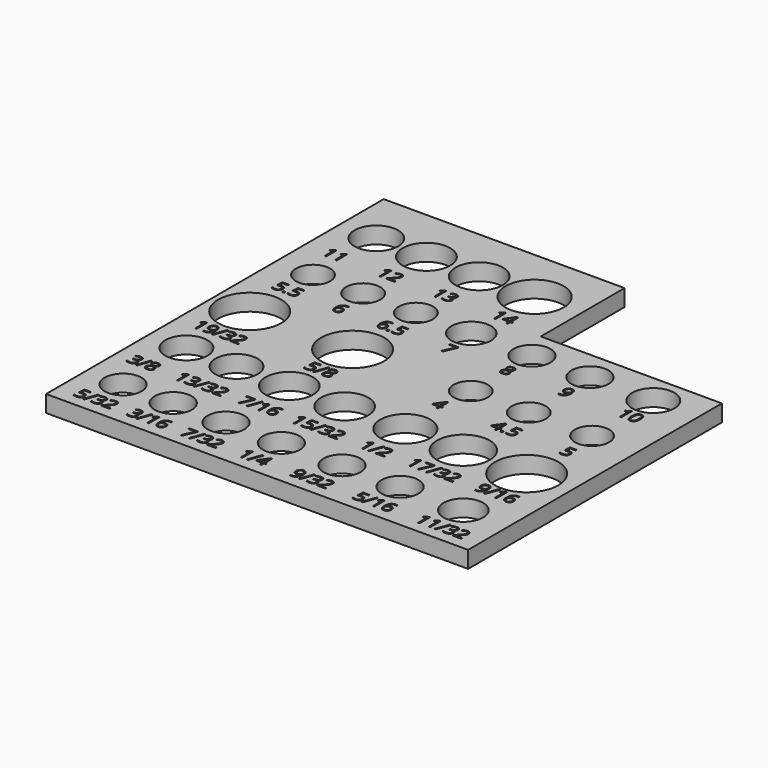
from build123d import *

# Parameters (mm, degrees)
F0_W         = 160
F0_H         = 160
F0_R         = 7
F0_R_2       = 8
F0_R_3       = 12
F0_R_4       = 9
F0_R_5       = 7.5
F0_R_6       = 9.5
F0_R_7       = 10
F0_R_8       = 6.5
F0_R_9       = 8.255
F0_R_10      = 11
F1_DEPTH     = 6.35
F2_TEXT_SIZE = 7.021965252
F3_DEPTH     = 2
F4_W         = 68.6776888743
F4_H         = 39.7198776901
F5_DEPTH     = 6.35


# Not quite as in the source:
# - Text() gives the source's letters only with a copy of the font that has no kerning and outlines rounded to 1/6400 em; it was checked with that copy


with BuildPart() as f1:
    # F0 (on Top) → F1 (new body)
    with BuildSketch(Plane.XY):
        Rectangle(F0_W, F0_H)
        with Locations((-66, -61)):
            Circle(F0_R, mode=Mode.SUBTRACT)
        with Locations((-47, -61)):
            Circle(F0_R, mode=Mode.SUBTRACT)
        with Locations((-27, -61)):
            Circle(F0_R, mode=Mode.SUBTRACT)
        with Locations((-6, -61)):
            Circle(F0_R, mode=Mode.SUBTRACT)
        with Locations((-66, -31)):
            Circle(F0_R_2, mode=Mode.SUBTRACT)
        with Locations((-47, -31)):
            Circle(F0_R_2, mode=Mode.SUBTRACT)
        with Locations((-66, -1)):
            Circle(F0_R_3, mode=Mode.SUBTRACT)
        with Locations((-27, -31)):
            Circle(F0_R_4, mode=Mode.SUBTRACT)
        with Locations((-6, -31)):
            Circle(F0_R_4, mode=Mode.SUBTRACT)
        with Locations((-27, -1)):
            Circle(F0_R_3, mode=Mode.SUBTRACT)
        with Locations((17, -61)):
            Circle(F0_R, mode=Mode.SUBTRACT)
        with Locations((39, -61)):
            Circle(F0_R, mode=Mode.SUBTRACT)
        with Locations((63, -61)):
            Circle(F0_R_5, mode=Mode.SUBTRACT)
        with Locations((17, -31)):
            Circle(F0_R_6, mode=Mode.SUBTRACT)
        with Locations((39, -31)):
            Circle(F0_R_7, mode=Mode.SUBTRACT)
        with Locations((63, -31)):
            Circle(F0_R_3, mode=Mode.SUBTRACT)
        with Locations((-66, 29)):
            Circle(F0_R_8, mode=Mode.SUBTRACT)
        with Locations((-47, 29)):
            Circle(F0_R_8, mode=Mode.SUBTRACT)
        with Locations((-27, 29)):
            Circle(F0_R_8, mode=Mode.SUBTRACT)
        with Locations((-6, 29)):
            Circle(F0_R_5, mode=Mode.SUBTRACT)
        with Locations((-66, 59)):
            Circle(F0_R_9, mode=Mode.SUBTRACT)
        with Locations((-47, 59)):
            Circle(F0_R_4, mode=Mode.SUBTRACT)
        with Locations((-27, 59)):
            Circle(F0_R_4, mode=Mode.SUBTRACT)
        with Locations((-6, 59)):
            Circle(F0_R_10, mode=Mode.SUBTRACT)
        with Locations((17, 0)):
            Circle(F0_R_8, mode=Mode.SUBTRACT)
        with Locations((39, 0)):
            Circle(F0_R_8, mode=Mode.SUBTRACT)
        with Locations((17, 29)):
            Circle(F0_R, mode=Mode.SUBTRACT)
        with Locations((39, 29)):
            Circle(F0_R, mode=Mode.SUBTRACT)
        with Locations((63, 0)):
            Circle(F0_R_8, mode=Mode.SUBTRACT)
        with Locations((63, 29)):
            Circle(F0_R_2, mode=Mode.SUBTRACT)
    extrude(amount=F1_DEPTH)

    # F2 (on face) → F3 (cut)
    with BuildSketch(Plane.XY.offset(6.35)):
        with Locations((-73.6421626061, -75.6910070777)):
            Text('5/32   3/16   7/32    1/4     9/32     5/16     11/32', F2_TEXT_SIZE, font='Open Sans', text_align=(TextAlign.LEFT, TextAlign.BOTTOM))
        with Locations((-75.046505779, -48.8898828626)):
            Text('3/8    13/32   7/16   15/32    1/2    17/32    9/16', F2_TEXT_SIZE, font='Open Sans', text_align=(TextAlign.LEFT, TextAlign.BOTTOM))
        with Locations((-73.7219527364, -19.5070735062)):
            Text('19/32             5/8', F2_TEXT_SIZE, font='Open Sans', text_align=(TextAlign.LEFT, TextAlign.BOTTOM))
        with Locations((13.2204908878, -14.8702124134)):
            Text('4          4.5         5', F2_TEXT_SIZE, font='Open Sans', text_align=(TextAlign.LEFT, TextAlign.BOTTOM))
        with Locations((-70.8629544824, 14.6579993889)):
            Text('5.5       6       6.5        7          8          9          10', F2_TEXT_SIZE, font='Open Sans', text_align=(TextAlign.LEFT, TextAlign.BOTTOM))
        with Locations((-72.7883409709, 40.5982108787)):
            Text('11       12       13        14', F2_TEXT_SIZE, font='Open Sans', text_align=(TextAlign.LEFT, TextAlign.BOTTOM))
    extrude(amount=-F3_DEPTH, mode=Mode.SUBTRACT)

    # F4 (on face) → F5 (cut, through all)
    with BuildSketch(Plane.XY.offset(6.35)):
        with Locations((45.6611555628, 60.140061155)):
            Rectangle(F4_W, F4_H)
    extrude(amount=-F5_DEPTH, mode=Mode.SUBTRACT)


solid = f1.part
